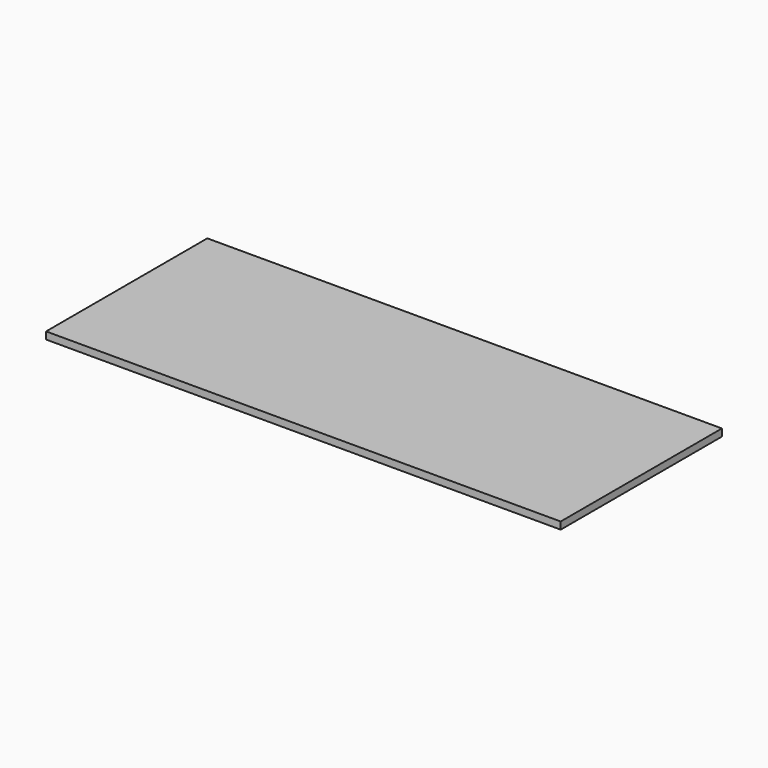
from build123d import *

# Parameters (mm, degrees)
F0_W     = 143
F0_H     = 56
F1_DEPTH = 2


# Not quite as in the source:
# - the program builds the solid bodies; features that only make, move or delete a surface that nothing else refers to are left out


with BuildPart() as f1:
    # F0 (on Top) → F1 (new body)
    with BuildSketch(Plane.XY):
        with Locations((71.5, 28)):
            Rectangle(F0_W, F0_H)
    extrude(amount=F1_DEPTH)


solid = f1.part
